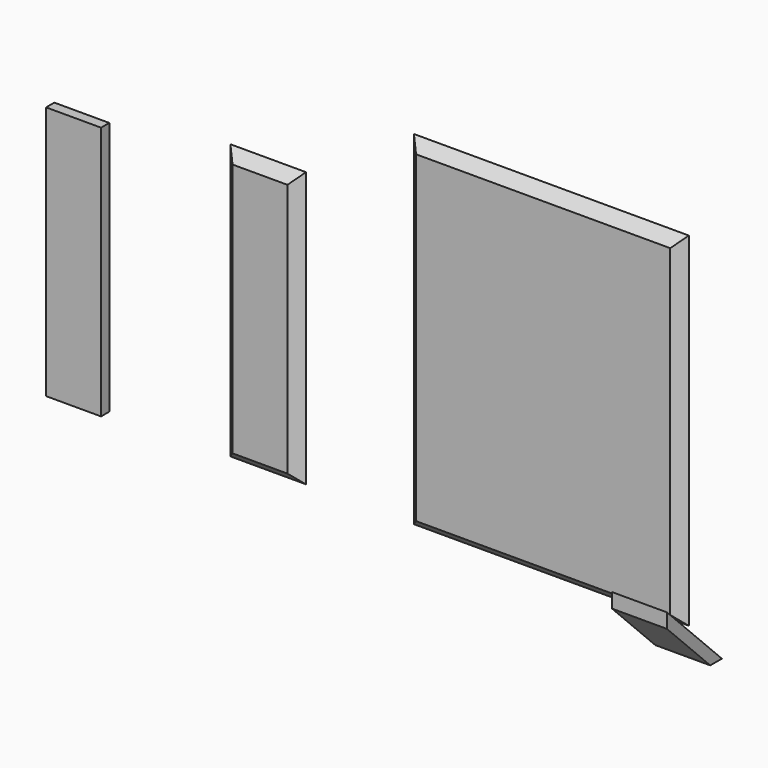
from build123d import *

# Parameters (mm, degrees)
F0_W      = 400
F0_H      = 500
F1_DEPTH  = 15
F2_W      = 110
F2_H      = 400
F3_DEPTH  = 15
F4_SIZE   = 14.99999
F4_2_SIZE = 14.99999
F5_W      = 80
F5_H      = 370
F6_DEPTH  = 15
F8_DEPTH  = 80


# Not quite as in the source:
# - a fillet or chamfer is up to 0.001 mm smaller than in the source, because OpenCascade refuses the exact size


with BuildPart() as f1:
    # F0 (on Front) → F1 (new body)
    with BuildSketch(Plane.XZ):
        with Locations((-200, 250)):
            Rectangle(F0_W, F0_H)
    extrude(amount=F1_DEPTH)

    # F4 (size 15 in the source; OpenCascade refuses exactly that, so slightly less here)
    f4_edges = [f1.edges().sort_by_distance(p)[0] for p in [
        (-200, -15, 0),
        (0, -15, 250),
        (-200, -15, 500),
        (-400, -15, 250),
    ]]
    chamfer(f4_edges, length=F4_SIZE)


with BuildPart() as f3:
    # F2 (on Front) → F3 (new body)
    with BuildSketch(Plane.XZ):
        with Locations((-612.1029348396, 200)):
            Rectangle(F2_W, F2_H)
    extrude(amount=F3_DEPTH)

    # F4#2 (size 15 in the source; OpenCascade refuses exactly that, so slightly less here)
    f4_2_edges = [f3.edges().sort_by_distance(p)[0] for p in [
        (-612.102935, -15, 0),
        (-557.102935, -15, 200),
        (-612.102935, -15, 400),
        (-667.102935, -15, 200),
    ]]
    chamfer(f4_2_edges, length=F4_2_SIZE)


with BuildPart() as f6:
    # F5 (on Front) → F6 (new body)
    with BuildSketch(Plane.XZ):
        with Locations((-883.413142176, 185)):
            Rectangle(F5_W, F5_H)
    extrude(amount=F6_DEPTH)


with BuildPart() as f8:
    # F7 (on Right) → F8 (new body)
    with BuildSketch(Plane.YZ):
        Polygon((-60.940527683, 0), (-39.7273242474, 0), (-139.7273242474, 100), (-139.7273242474, 78.7867965644), align=None)
    extrude(amount=F8_DEPTH)


solid = Compound([f1.part, f3.part, f6.part, f8.part])
